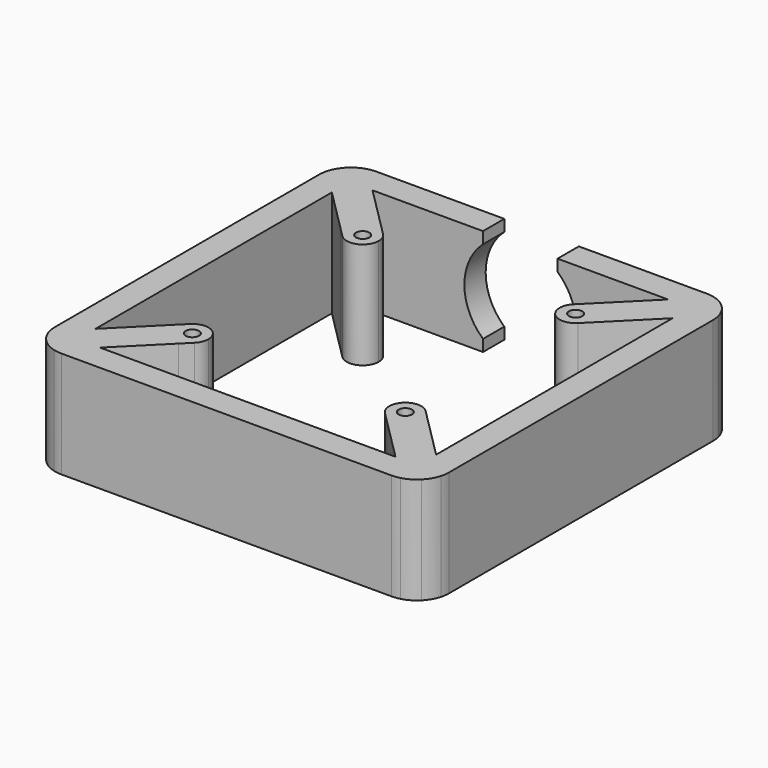
from build123d import *

# Parameters (mm, degrees)
F1_DEPTH = 20
F3_DEPTH = 25
F6_D     = 2.5


# Not quite as in the source:
# - a feature names something its author has since deleted; it is built from what else it names


with BuildPart() as f1:
    # F0 (on Top) → F1 (new body)
    with BuildSketch(Plane.XY):
        with BuildLine():
            Line((0, 68), (0, 6))
            ThreePointArc((0, 6), (0.0513308318, 5.2168428467), (0.2044450423, 4.4470857294))
            Line((0.2044450423, 4.4470857294), (5, 9.2426406871))
            Line((5, 9.2426406871), (5, 24.5))
            Line((5, 24.5), (5, 49))
            Line((5, 49), (5, 64.7573593129))
            Line((5, 64.7573593129), (0.2044450423, 69.5529142706))
            ThreePointArc((0.2044450423, 69.5529142706), (0.0513308318, 68.7831571533), (0, 68))
        make_face()
        with BuildLine():
            Line((5, 9.2426406871), (0.2044450423, 4.4470857294))
            ThreePointArc((0.2044450423, 4.4470857294), (0.8038475773, 3), (1.7573593129, 1.7573593129))
            Line((1.7573593129, 1.7573593129), (5.2928932188, 5.2928932188))
            ThreePointArc((5.2928932188, 5.2928932188), (5.0761204675, 5.6173165676), (5, 6))
            Line((5, 6), (5, 9.2426406871))
        make_face()
        with BuildLine():
            ThreePointArc((1.7573593129, 72.2426406871), (0.8038475773, 71), (0.2044450423, 69.5529142706))
            Line((0.2044450423, 69.5529142706), (5, 64.7573593129))
            Line((5, 64.7573593129), (5, 68))
            ThreePointArc((5, 68), (5.0761204675, 68.3826834324), (5.2928932188, 68.7071067812))
            Line((5.2928932188, 68.7071067812), (1.7573593129, 72.2426406871))
        make_face()
        with BuildLine():
            Line((5.2928932188, 5.2928932188), (1.7573593129, 1.7573593129))
            ThreePointArc((1.7573593129, 1.7573593129), (3, 0.8038475773), (4.4470857294, 0.2044450423))
            Line((4.4470857294, 0.2044450423), (9.2426406871, 5))
            Line((9.2426406871, 5), (6, 5))
            ThreePointArc((6, 5), (5.6173165676, 5.0761204675), (5.2928932188, 5.2928932188))
        make_face()
        with BuildLine():
            Line((14.8786796564, 19.1213203436), (5, 9.2426406871))
            Line((5, 9.2426406871), (5, 6))
            ThreePointArc((5, 6), (5.0761204675, 5.6173165676), (5.2928932188, 5.2928932188))
            Line((5.2928932188, 5.2928932188), (14.8786796564, 14.8786796564))
            ThreePointArc((14.8786796564, 14.8786796564), (14, 17), (14.8786796564, 19.1213203436))
        make_face()
        with BuildLine():
            ThreePointArc((4.4470857294, 73.7955549577), (3, 73.1961524227), (1.7573593129, 72.2426406871))
            Line((1.7573593129, 72.2426406871), (5.2928932188, 68.7071067812))
            ThreePointArc((5.2928932188, 68.7071067812), (5.6173165676, 68.9238795325), (6, 69))
            Line((6, 69), (9.2426406871, 69))
            Line((9.2426406871, 69), (4.4470857294, 73.7955549577))
        make_face()
        with BuildLine():
            Line((5, 68), (5, 64.7573593129))
            Line((5, 64.7573593129), (13.1819805153, 56.5753787975))
            Line((13.1819805153, 56.5753787975), (14.8786796564, 54.8786796564))
            ThreePointArc((14.8786796564, 54.8786796564), (14, 57), (14.8786796564, 59.1213203436))
            Line((14.8786796564, 59.1213203436), (5.2928932188, 68.7071067812))
            ThreePointArc((5.2928932188, 68.7071067812), (5.0761204675, 68.3826834324), (5, 68))
        make_face()
        with BuildLine():
            Line((9.2426406871, 5), (4.4470857294, 0.2044450423))
            ThreePointArc((4.4470857294, 0.2044450423), (5.2168428467, 0.0513308318), (6, 0))
            Line((6, 0), (37, 0))
            Line((37, 0), (68, 0))
            ThreePointArc((68, 0), (68.7831571533, 0.0513308318), (69.5529142706, 0.2044450423))
            Line((69.5529142706, 0.2044450423), (64.7573593129, 5))
            Line((64.7573593129, 5), (37, 5))
            Line((37, 5), (30, 5))
            Line((30, 5), (9.2426406871, 5))
        make_face()
        with BuildLine():
            Line((14.8786796564, 14.8786796564), (5.2928932188, 5.2928932188))
            ThreePointArc((5.2928932188, 5.2928932188), (5.6173165676, 5.0761204675), (6, 5))
            Line((6, 5), (9.2426406871, 5))
            Line((9.2426406871, 5), (17.4246212025, 13.1819805153))
            Line((17.4246212025, 13.1819805153), (19.1213203436, 14.8786796564))
            ThreePointArc((19.1213203436, 14.8786796564), (17, 14), (14.8786796564, 14.8786796564))
        make_face()
        with BuildLine():
            ThreePointArc((20, 17), (18.1480502971, 19.7716385975), (14.8786796564, 19.1213203436))
            ThreePointArc((14.8786796564, 19.1213203436), (14, 17), (14.8786796564, 14.8786796564))
            ThreePointArc((14.8786796564, 14.8786796564), (17, 14), (19.1213203436, 14.8786796564))
            ThreePointArc((19.1213203436, 14.8786796564), (19.7716385975, 15.8519497029), (20, 17))
        make_face()
        with BuildLine():
            ThreePointArc((6, 74), (5.2168428467, 73.9486691682), (4.4470857294, 73.7955549577))
            Line((4.4470857294, 73.7955549577), (9.2426406871, 69))
            Line((9.2426406871, 69), (30, 69))
            Line((30, 69), (30, 74))
            Line((30, 74), (6, 74))
        make_face()
        with BuildLine():
            ThreePointArc((6, 69), (5.6173165676, 68.9238795325), (5.2928932188, 68.7071067812))
            Line((5.2928932188, 68.7071067812), (14.8786796564, 59.1213203436))
            ThreePointArc((14.8786796564, 59.1213203436), (17, 60), (19.1213203436, 59.1213203436))
            Line((19.1213203436, 59.1213203436), (17.4246212025, 60.8180194847))
            Line((17.4246212025, 60.8180194847), (9.2426406871, 69))
            Line((9.2426406871, 69), (6, 69))
        make_face()
        with BuildLine():
            ThreePointArc((19.1213203436, 59.1213203436), (17, 60), (14.8786796564, 59.1213203436))
            ThreePointArc((14.8786796564, 59.1213203436), (14, 57), (14.8786796564, 54.8786796564))
            ThreePointArc((14.8786796564, 54.8786796564), (18.1480502971, 54.2283614025), (20, 57))
            ThreePointArc((20, 57), (19.7716385975, 58.1480502971), (19.1213203436, 59.1213203436))
        make_face()
        with BuildLine():
            Line((64.7573593129, 5), (69.5529142706, 0.2044450423))
            ThreePointArc((69.5529142706, 0.2044450423), (71, 0.8038475773), (72.2426406871, 1.7573593129))
            Line((72.2426406871, 1.7573593129), (68.7071067812, 5.2928932188))
            ThreePointArc((68.7071067812, 5.2928932188), (68.3826834324, 5.0761204675), (68, 5))
            Line((68, 5), (64.7573593129, 5))
        make_face()
        with BuildLine():
            Line((56.5753787975, 13.1819805153), (64.7573593129, 5))
            Line((64.7573593129, 5), (68, 5))
            ThreePointArc((68, 5), (68.3826834324, 5.0761204675), (68.7071067812, 5.2928932188))
            Line((68.7071067812, 5.2928932188), (59.1213203436, 14.8786796564))
            ThreePointArc((59.1213203436, 14.8786796564), (57, 14), (54.8786796564, 14.8786796564))
            Line((54.8786796564, 14.8786796564), (56.5753787975, 13.1819805153))
        make_face()
        with BuildLine():
            Line((68.7071067812, 5.2928932188), (72.2426406871, 1.7573593129))
            ThreePointArc((72.2426406871, 1.7573593129), (73.1961524227, 3), (73.7955549577, 4.4470857294))
            Line((73.7955549577, 4.4470857294), (69, 9.2426406871))
            Line((69, 9.2426406871), (69, 6))
            ThreePointArc((69, 6), (68.9238795325, 5.6173165676), (68.7071067812, 5.2928932188))
        make_face()
        with BuildLine():
            Line((69, 9.2426406871), (73.7955549577, 4.4470857294))
            ThreePointArc((73.7955549577, 4.4470857294), (73.9486691682, 5.2168428467), (74, 6))
            Line((74, 6), (74, 68))
            ThreePointArc((74, 68), (73.9486691682, 68.7831571533), (73.7955549577, 69.5529142706))
            Line((73.7955549577, 69.5529142706), (69, 64.7573593129))
            Line((69, 64.7573593129), (69, 49))
            Line((69, 49), (69, 24.5))
            Line((69, 24.5), (69, 9.2426406871))
        make_face()
        with BuildLine():
            Line((59.1213203436, 14.8786796564), (68.7071067812, 5.2928932188))
            ThreePointArc((68.7071067812, 5.2928932188), (68.9238795325, 5.6173165676), (69, 6))
            Line((69, 6), (69, 9.2426406871))
            Line((69, 9.2426406871), (59.1213203436, 19.1213203436))
            ThreePointArc((59.1213203436, 19.1213203436), (59.7716385975, 18.1480502971), (60, 17))
            ThreePointArc((60, 17), (59.7716385975, 15.8519497029), (59.1213203436, 14.8786796564))
        make_face()
        with BuildLine():
            ThreePointArc((59.1213203436, 19.1213203436), (54.8786796564, 19.1213203436), (54.8786796564, 14.8786796564))
            ThreePointArc((54.8786796564, 14.8786796564), (57, 14), (59.1213203436, 14.8786796564))
            ThreePointArc((59.1213203436, 14.8786796564), (59.7716385975, 15.8519497029), (60, 17))
            ThreePointArc((60, 17), (59.7716385975, 18.1480502971), (59.1213203436, 19.1213203436))
        make_face()
        with BuildLine():
            Line((69, 64.7573593129), (73.7955549577, 69.5529142706))
            ThreePointArc((73.7955549577, 69.5529142706), (73.1961524227, 71), (72.2426406871, 72.2426406871))
            Line((72.2426406871, 72.2426406871), (68.7071067812, 68.7071067812))
            ThreePointArc((68.7071067812, 68.7071067812), (68.9238795325, 68.3826834324), (69, 68))
            Line((69, 68), (69, 64.7573593129))
        make_face()
        with BuildLine():
            Line((68.7071067812, 68.7071067812), (72.2426406871, 72.2426406871))
            ThreePointArc((72.2426406871, 72.2426406871), (71, 73.1961524227), (69.5529142706, 73.7955549577))
            Line((69.5529142706, 73.7955549577), (64.7573593129, 69))
            Line((64.7573593129, 69), (68, 69))
            ThreePointArc((68, 69), (68.3826834324, 68.9238795325), (68.7071067812, 68.7071067812))
        make_face()
        with BuildLine():
            Line((59.1213203436, 54.8786796564), (69, 64.7573593129))
            Line((69, 64.7573593129), (69, 68))
            ThreePointArc((69, 68), (68.9238795325, 68.3826834324), (68.7071067812, 68.7071067812))
            Line((68.7071067812, 68.7071067812), (59.1213203436, 59.1213203436))
            ThreePointArc((59.1213203436, 59.1213203436), (59.7716385975, 58.1480502971), (60, 57))
            ThreePointArc((60, 57), (59.7716385975, 55.8519497029), (59.1213203436, 54.8786796564))
        make_face()
        with BuildLine():
            Line((64.7573593129, 69), (69.5529142706, 73.7955549577))
            ThreePointArc((69.5529142706, 73.7955549577), (68.7831571533, 73.9486691682), (68, 74))
            Line((68, 74), (44, 74))
            Line((44, 74), (44, 69))
            Line((44, 69), (64.7573593129, 69))
        make_face()
        with BuildLine():
            Line((59.1213203436, 59.1213203436), (68.7071067812, 68.7071067812))
            ThreePointArc((68.7071067812, 68.7071067812), (68.3826834324, 68.9238795325), (68, 69))
            Line((68, 69), (64.7573593129, 69))
            Line((64.7573593129, 69), (56.5753787975, 60.8180194847))
            Line((56.5753787975, 60.8180194847), (54.8786796564, 59.1213203436))
            ThreePointArc((54.8786796564, 59.1213203436), (57, 60), (59.1213203436, 59.1213203436))
        make_face()
        with BuildLine():
            ThreePointArc((54.8786796564, 59.1213203436), (54.8786796564, 54.8786796564), (59.1213203436, 54.8786796564))
            ThreePointArc((59.1213203436, 54.8786796564), (59.7716385975, 55.8519497029), (60, 57))
            ThreePointArc((60, 57), (59.7716385975, 58.1480502971), (59.1213203436, 59.1213203436))
            ThreePointArc((59.1213203436, 59.1213203436), (57, 60), (54.8786796564, 59.1213203436))
        make_face()
    extrude(amount=F1_DEPTH)


with BuildPart() as f3:
    # F2 (on face) → F3 (new body)
    with BuildSketch(Plane(origin=(0, 74, 0), x_dir=(-1, 0, 0), z_dir=(0, 1, 0))):
        with BuildLine():
            ThreePointArc((-26.5, 10), (-37, 20.5), (-47.5, 10))
            Line((-47.5, 10), (-26.5, 10))
        make_face()
        with BuildLine():
            Line((-26.5, 10), (-47.5, 10))
            ThreePointArc((-47.5, 10), (-37, -0.5), (-26.5, 10))
        make_face()
    extrude(amount=-F3_DEPTH)


with BuildPart() as f1_1:
    add(f1.part)

    # F4: cut F3
    add(f3.part, mode=Mode.SUBTRACT)

    # F6 (through all)
    with Locations(Plane.XY.offset(20)):
        with Locations((17, 57), (57, 57), (57, 17), (17, 17)):
            Hole(F6_D / 2)


solid = f1_1.part
